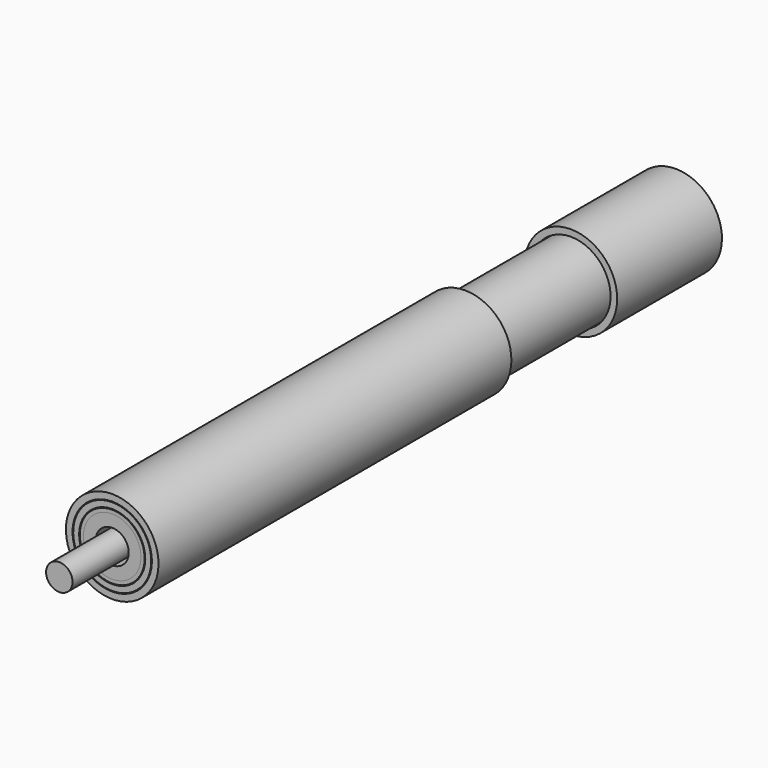
from build123d import *

# Parameters (mm, degrees)
F0_W   = 5
F0_H   = 0.9
F0_W_2 = 19.8
F0_H_2 = 1
F0_W_3 = 8


# Not quite as in the source:
# - ends of sketch curves that miss each other by under 0.0002 mm in the source are joined
# - the dataset's text gives a spline's control points without its knots; the knots are read off the source's solid


with BuildPart() as f1:
    # F0 (on Right) → F1 (revolve)
    with BuildSketch(Plane.YZ):
        Polygon((-10, 2), (-10, 0), (109.9562048912, 0), (109.9562048912, 2), (90, 2), (30, 2), align=None)
    revolve(axis=Axis((0, 49.9781024456, 0), (0, 1, 0)))


with BuildPart() as f1b:
    # F0 (on Right) → F1, piece 2 (revolve)
    with BuildSketch(Plane.YZ):
        with Locations((2.5, 5.45)):
            Rectangle(F0_W, F0_H)
    revolve(axis=Axis((0, 49.9781024456, 0), (0, 1, 0)))


with BuildPart() as f1c:
    # F0 (on Right) → F1, piece 3 (revolve)
    with BuildSketch(Plane.YZ):
        with BuildLine():
            Line((22.7739673619, 2.5), (22.7739673619, 3.5))
            add(Edge.make_bspline(
                [(5, 4.35), (7.5, 4.35), (7.6531279723, 6.4931177104), (18.1980438679, 4.4662913108), (22.7739673619, 3.5)],
                knots=[0, 0, 0, 0, 0.3343138665, 0.7023845554, 0.7023845554, 0.7023845554, 0.7023845554], degree=3))
            Line((5, 4.35), (0, 4.35))
            Line((0, 4.35), (0, 2.5))
            Line((0, 2.5), (22.7739673619, 2.5))
        make_face()
    revolve(axis=Axis((0, 49.9781024456, 0), (0, 1, 0)))


with BuildPart() as f1d:
    # F0 (on Right) → F1, piece 4 (revolve)
    with BuildSketch(Plane.YZ):
        with BuildLine():
            Line((18.6169619347, 5.9), (18.6169619347, 4.9))
            add(Edge.make_bspline(
                [(18.6169619347, 4.9), (19.1077885857, 4.806759458), (20.4281555034, 4.5492492317), (22.5501965572, 4.1125672039), (24.8517755762, 3.6192994533), (26.5480859484, 3.2490049406), (27.4234542671, 3.0591169406), (27.6972536968, 3.0001393389), (27.6979005808, 2.9999999997)],
                knots=[0.5922816967, 0.5922816967, 0.5922816967, 0.5922816967, 0.6297531173, 0.692728429, 0.7557037407, 0.8186790524, 0.8501667083, 0.8502412898, 0.8502412898, 0.8502412898, 0.8502412898], degree=3))
            Line((27.6979005808, 2.9999999997), (32.7739673619, 3))
            Line((32.7739673619, 3), (32.7739673619, 4.9))
            Line((32.7739673619, 4.9), (24.7739673619, 4.9))
            Line((24.7739673619, 4.9), (24.7739673619, 5))
            Line((24.7739673619, 5), (24.7739673619, 5.9))
            Line((24.7739673619, 5.9), (18.6169619347, 5.9))
        make_face()
    revolve(axis=Axis((0, 49.9781024456, 0), (0, 1, 0)))


with BuildPart() as f1e:
    # F0 (on Right) → F1, piece 5 (revolve)
    with BuildSketch(Plane.YZ):
        Polygon((91.7, 5), (91.7, 5.9), (52.7739673619, 5.9), (52.7739673619, 5), (86.7, 5), align=None)
    revolve(axis=Axis((0, 49.9781024456, 0), (0, 1, 0)))


with BuildPart() as f1f:
    # F0 (on Right) → F1, piece 6 (revolve)
    with BuildSketch(Plane.YZ):
        with Locations((96.6, 6.5)):
            Rectangle(F0_W_2, F0_H_2)
    revolve(axis=Axis((0, 49.9781024456, 0), (0, 1, 0)))


with BuildPart() as f2:
    # F0 (on Right) → F2 (revolve)
    with BuildSketch(Plane.YZ):
        with BuildLine():
            add(Edge.make_bspline(
                [(22.7739673619, 3.5), (26.4739781102, 2.7186739484), (29.5529192669, 2), (30, 2)],
                knots=[0.7023845554, 0.7023845554, 0.7023845554, 0.7023845554, 1, 1, 1, 1], degree=3))
            Line((30, 2), (90, 2))
            Line((90, 2), (95, 2.5))
            Line((95, 2.5), (105, 2.5))
            ThreePointArc((105, 2.5), (106.5, 4), (105, 5.5))
            Line((105, 5.5), (95, 5.5))
            ThreePointArc((95, 5.5), (94.7878679656, 5.4121320344), (94.7, 5.2))
            ThreePointArc((94.7, 5.2), (94.7878679656, 4.9878679656), (95, 4.9))
            Line((95, 4.9), (105, 4.9))
            ThreePointArc((105, 4.9), (105.9, 4), (105, 3.1))
            Line((105, 3.1), (95, 3.1))
            Line((95, 3.1), (90, 2.5500482411))
            Line((90, 2.5500482411), (30, 2.5500482411))
            add(Edge.make_bspline(
                [(27.6979005808, 2.9999999997), (27.9703626299, 2.9413115213), (28.4793254325, 2.8325626294), (29.0114292656, 2.7225539191), (29.3664304036, 2.6526113095), (29.5946052051, 2.6099185693), (29.7816205477, 2.5777310728), (29.8990378353, 2.5603998228), (29.9653790868, 2.5526565183), (29.9899666449, 2.5505485906), (29.9988060823, 2.5501172971), (30, 2.5500482411)],
                knots=[0.8502412898, 0.8502412898, 0.8502412898, 0.8502412898, 0.8816543642, 0.91314202, 0.928885848, 0.9446296759, 0.9603735038, 0.9761173318, 0.9839892457, 0.9918611597, 0.9948060117, 0.9948060117, 0.9948060117, 0.9948060117], degree=3))
            add(Edge.make_bspline(
                [(18.6169619937, 4.9000003106), (19.1077885857, 4.806759458), (20.4281555034, 4.5492492317), (22.5501965572, 4.1125672039), (24.8517755762, 3.6192994533), (26.5480859484, 3.2490049406), (27.4234542671, 3.0591169406), (27.6972536968, 3.0001393389), (27.6979005808, 2.9999999997)],
                knots=[0.5922816967, 0.5922816967, 0.5922816967, 0.5922816967, 0.6297531173, 0.692728429, 0.7557037407, 0.8186790524, 0.8501667083, 0.8502412898, 0.8502412898, 0.8502412898, 0.8502412898], degree=3))
            add(Edge.make_bspline(
                [(10.3135561122, 6.0000216452), (10.557163937, 6.0000212859), (11.3664076489, 5.9760546241), (12.9603330043, 5.8289629435), (15.1899505113, 5.5127649815), (17.1267180593, 5.1790901518), (18.2828943815, 4.9634621308), (18.6169619937, 4.9000003106)],
                knots=[0.3481533145, 0.3481533145, 0.3481533145, 0.3481533145, 0.3778518704, 0.4408271821, 0.5038024938, 0.5667778055, 0.5922816967, 0.5922816967, 0.5922816967, 0.5922816967], degree=3))
            add(Edge.make_bspline(
                [(5, 4.9), (5.4427474864, 4.9), (6.143703495, 4.9679889371), (6.8690177635, 5.1830093381), (7.5413553934, 5.4778384291), (8.2327974026, 5.7429025369), (8.9291678865, 5.9005200323), (9.536432354, 5.9795606064), (10.0269834642, 5.9995036631), (10.2988806925, 6.0000216668), (10.3135561122, 6.0000216452)],
                knots=[0, 0, 0, 0, 0.0629753117, 0.1259506235, 0.1889259352, 0.2519012469, 0.2833889028, 0.3148765586, 0.3463642145, 0.3481533145, 0.3481533145, 0.3481533145, 0.3481533145], degree=3))
            Line((5, 4.9), (0, 4.9))
            Line((0, 4.9), (0, 4.35))
            Line((0, 4.35), (5, 4.35))
            add(Edge.make_bspline(
                [(5, 4.35), (7.5, 4.35), (7.6531279723, 6.4931177104), (18.1980438679, 4.4662913108), (22.7739673619, 3.5)],
                knots=[0, 0, 0, 0, 0.3343138665, 0.7023845554, 0.7023845554, 0.7023845554, 0.7023845554], degree=3))
        make_face()
    revolve(axis=Axis((0, 49.9781024456, 0), (0, 1, 0)))


with BuildPart() as f2b:
    # F0 (on Right) → F2, piece 2 (revolve)
    with BuildSketch(Plane.YZ):
        with Locations((28.7739673619, 5.45)):
            Rectangle(F0_W_3, F0_H)
    revolve(axis=Axis((0, 49.9781024456, 0), (0, 1, 0)))


with BuildPart() as f3:
    # F0 (on Right) → F3 (revolve)
    with BuildSketch(Plane.YZ):
        Polygon((0, 6), (10.3135561122, 6), (66.7, 6), (66.7, 7), (0, 7), align=None)
    revolve(axis=Axis((0, 49.9781024456, 0), (0, 1, 0)))


with BuildPart() as f3b:
    # F0 (on Right) → F3, piece 2 (revolve)
    with BuildSketch(Plane.YZ):
        with BuildLine():
            Line((94.7, 4.9), (94.7, 5.2))
            Line((94.7, 5.2), (94.7, 5.9))
            Line((94.7, 5.9), (91.7, 5.9))
            Line((91.7, 5.9), (91.7, 5))
            Line((91.7, 5), (86.7, 5))
            Line((86.7, 5), (86.7, 3.1))
            Line((86.7, 3.1), (95, 3.1))
            Line((95, 3.1), (105, 3.1))
            ThreePointArc((105, 3.1), (105.9, 4), (105, 4.9))
            Line((105, 4.9), (95, 4.9))
            Line((95, 4.9), (94.7, 4.9))
        make_face()
    revolve(axis=Axis((0, 49.9781024456, 0), (0, 1, 0)))


solid = Compound([f1.part, f1b.part, f1c.part, f1d.part, f1e.part, f1f.part, f2.part, f2b.part, f3.part, f3b.part])
